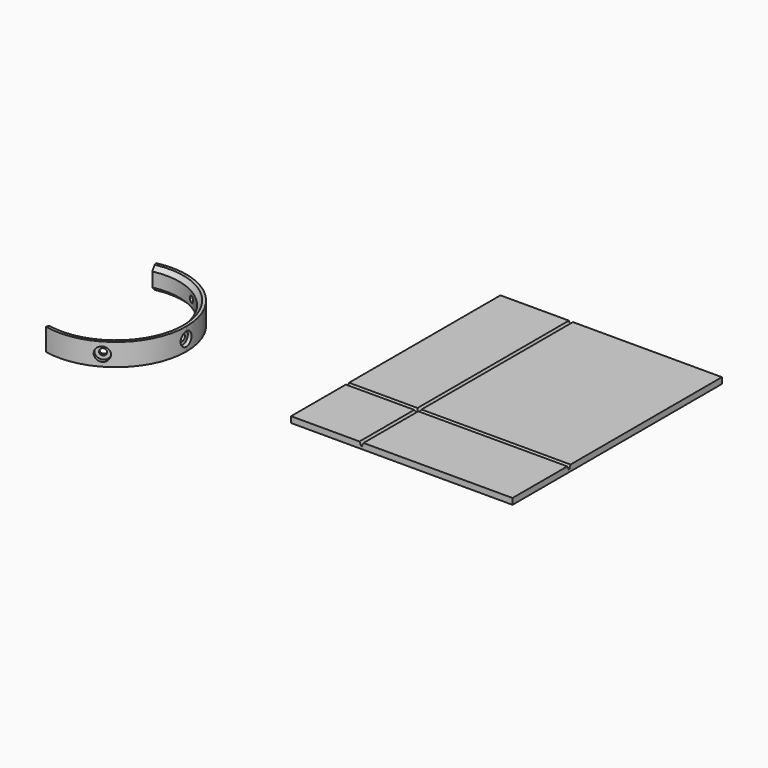
from build123d import *

# Parameters (mm, degrees)
F0_W           = 110
F0_H           = 130
F0_W_2         = 80
F0_H_2         = 100
F1_DEPTH       = 3
F3_DEPTH       = 140
F5_DEPTH       = 120
F7_R           = 35
F7_R_2         = 31.5
F8_DEPTH       = 5.5
F9_W           = 2.7181416105
F9_H           = 1.6
F15_ANGLE_BACK = 78
F15_ANGLE      = 156


# Not quite as in the source:
# - a feature names something its author has since deleted; it is built from what else it names


with BuildPart() as f1:
    # F0 (on Top) → F1 (new body)
    with BuildSketch(Plane.XY):
        with Locations((20, 30)):
            Rectangle(F0_W, F0_H)
        with Locations((20, 30)):
            Rectangle(F0_W_2, F0_H_2, mode=Mode.SUBTRACT)
        with Locations((20, 30)):
            Rectangle(F0_W_2, F0_H_2)
    extrude(amount=F1_DEPTH)

    # F2 (on face) → F3 (cut)
    with BuildSketch(Plane.XZ.offset(35)):
        Polygon((1, 3), (-1, 3), (0, 1), align=None)
    extrude(amount=-F3_DEPTH, mode=Mode.SUBTRACT)

    # F4 (on face) → F5 (cut)
    with BuildSketch(Plane.YZ.offset(75)):
        Polygon((1, 3), (-1, 3), (0, 1), align=None)
    extrude(amount=-F5_DEPTH, mode=Mode.SUBTRACT)


with BuildPart() as f8:
    # F7 (on offset) → F8 (new body, symmetric)
    with BuildSketch(Plane.XY.offset(-3.5)):
        with Locations((-150, 0)):
            Circle(F7_R)
        with Locations((-150, 0)):
            Circle(F7_R_2, mode=Mode.SUBTRACT)
    extrude(amount=F8_DEPTH, both=True)

    # F9 (on offset) → F10 (revolve, cut)
    with BuildSketch(Plane.XY.offset(-3.5)):
        Polygon((-132.0531194037, -31.0849090301), (-133.5, -28.5788383249), (-134.8856406461, -29.3788383249), (-136.4444863729, -30.2788383249), (-134.9976057766, -32.7849090301), align=None)
        Polygon((-134.8856406461, -29.3788383249), (-133.5, -28.5788383249), (-134.8590708053, -26.2248586391), (-136.2447114513, -27.0248586391), align=None)
    revolve(axis=Axis((-118.5595137524, -54.4565195956, -3.5), (0.5, -0.8660254038, 0)), mode=Mode.SUBTRACT)

    # F9 (on offset) → F11 (revolve, cut)
    with BuildSketch(Plane.XY.offset(-3.5)):
        Polygon((-114.1062388075, 0), (-117, 0), (-117, -1.6), (-117, -3.4), (-114.1062388075, -3.4), align=None)
        with Locations((-118.3590708053, -0.8)):
            Rectangle(F9_W, F9_H)
    revolve(axis=Axis((-87.1190275047, 0, -3.5), (1, 0, 0)), mode=Mode.SUBTRACT)

    # F9 (on offset) → F12 (revolve, cut)
    with BuildSketch(Plane.XY.offset(-3.5)):
        Polygon((-132.0531194037, 31.0849090301), (-133.5, 28.5788383249), (-132.1143593539, 27.7788383249), (-130.5555136271, 26.8788383249), (-129.1086330309, 29.3849090301), align=None)
        Polygon((-132.1143593539, 27.7788383249), (-133.5, 28.5788383249), (-134.8590708053, 26.2248586391), (-133.4734301592, 25.4248586391), align=None)
    revolve(axis=Axis((-118.5595137524, 54.4565195956, -3.5), (0.5, 0.8660254038, 0)), mode=Mode.SUBTRACT)

    # F9 (on offset) → F13 (revolve, cut)
    with BuildSketch(Plane.XY.offset(-3.5)):
        Polygon((-167.9468805963, -31.0849090301), (-166.5, -28.5788383249), (-167.8856406461, -27.7788383249), (-169.4444863729, -26.8788383249), (-170.8913669691, -29.3849090301), align=None)
        Polygon((-167.8856406461, -27.7788383249), (-166.5, -28.5788383249), (-165.1409291947, -26.2248586391), (-166.5265698408, -25.4248586391), align=None)
    revolve(axis=Axis((-181.4404862476, -54.4565195956, -3.5), (-0.5, -0.8660254038, 0)), mode=Mode.SUBTRACT)

    # F14 (on Front) → F15 (revolve, cut)
    with BuildSketch(Plane.XZ, mode=Mode.PRIVATE) as f15_sk:
        Polygon((-185, 0), (-185, -7), (-185, -9), (-183.5, -9), (-181.5, -7), (-181.5, 0), (-183.5, 2), (-185, 2), align=None)
    revolve(f15_sk.sketch.rotate(Axis((-150, 0, -3.5), (0, 0, 1)), -F15_ANGLE_BACK), axis=Axis((-150, 0, -3.5), (0, 0, 1)), revolution_arc=F15_ANGLE, mode=Mode.SUBTRACT)

    # F14 (on Front) → F16 (revolve, cut)
    with BuildSketch(Plane.XZ):
        Polygon((-181.5, 2), (-183.5, 2), (-181.5, 0), align=None)
        Polygon((-181.5, -7), (-183.5, -9), (-181.5, -9), align=None)
    revolve(axis=Axis((-150, 0, -3.5), (0, 0, 1)), mode=Mode.SUBTRACT)


solid = Compound([f1.part, f8.part])
